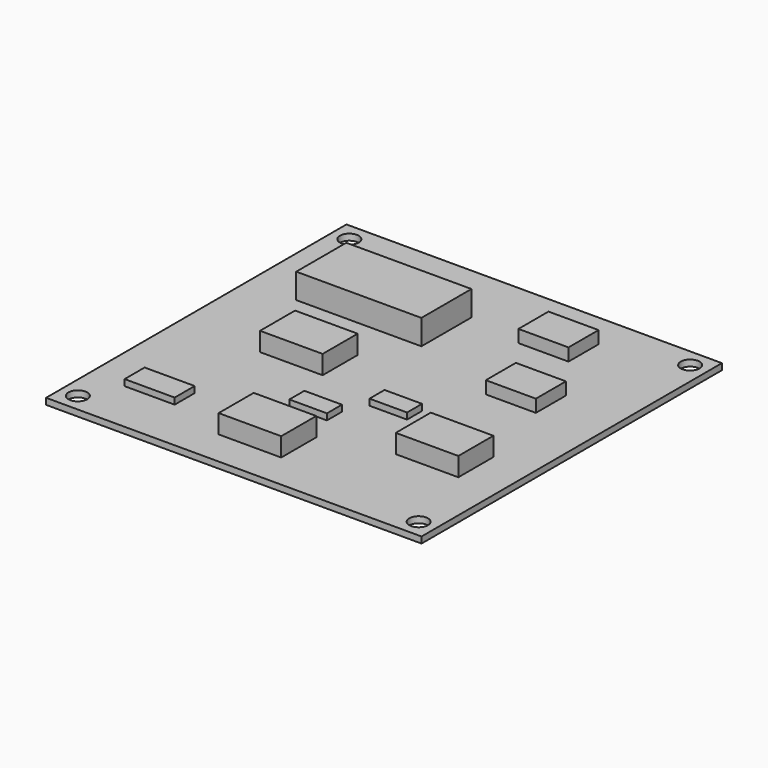
from build123d import *

# Parameters (mm, degrees)
F0_W      = 4
F0_H      = 2
F0_W_2    = 5
F0_H_2    = 3.5
F0_W_3    = 3
F0_H_3    = 1.5
F0_R      = 0.75
F0_W_4    = 10
F0_H_4    = 5
F0_H_5    = 3
F1_DEPTH  = 0.5
F2_DEPTH  = 0.5
F7_DEPTH  = 2
F8_DEPTH  = 1.5
F9_DEPTH  = 1
F10_DEPTH = 0.5


# Not quite as in the source:
# - the program builds the solid bodies; features that only make, move or delete a surface that nothing else refers to are left out


with BuildPart() as f1:
    # F0 (on Top) → F1 (new body)
    with BuildSketch(Plane.XY):
        Polygon((15, 15), (0, 15), (-15, 15), (-15, 0), (-15, -15), (15, -15), (15, 0), align=None)
        with Locations((-10.1540855616, -9.7154753059)):
            Rectangle(F0_W, F0_H, mode=Mode.SUBTRACT)
        with Locations((-1.0007002298, -10.3894498274)):
            Rectangle(F0_W_2, F0_H_2, mode=Mode.SUBTRACT)
        with Locations((-0.9053347297, -5.6935508102)):
            Rectangle(F0_W_3, F0_H_3, mode=Mode.SUBTRACT)
        with Locations((-5.9298439324, -0.0930169439)):
            Rectangle(F0_W_2, F0_H_2, mode=Mode.SUBTRACT)
        with Locations((2.9284434728, -2.4834803706)):
            Rectangle(F0_W_3, F0_H_3, mode=Mode.SUBTRACT)
        with Locations((9.2957332358, -5.5698433965)):
            Rectangle(F0_W_2, F0_H_2, mode=Mode.SUBTRACT)
        with Locations((-13.6142675997, 13.55786765)):
            Circle(F0_R, mode=Mode.SUBTRACT)
        with Locations((-6.0587198287, 7.557784263)):
            Rectangle(F0_W_4, F0_H_4, mode=Mode.SUBTRACT)
        with Locations((8.1385142617, 3.9959300905)):
            Rectangle(F0_W, F0_H_5, mode=Mode.SUBTRACT)
        with Locations((5.4001008607, 10.6776582673)):
            Rectangle(F0_W, F0_H_5, mode=Mode.SUBTRACT)
        with Locations((-6.0587198287, 7.557784263)):
            Rectangle(F0_W_4, F0_H_4)
        with Locations((-5.9298439324, -0.0930169439)):
            Rectangle(F0_W_2, F0_H_2)
        with Locations((-10.1540855616, -9.7154753059)):
            Rectangle(F0_W, F0_H)
        with Locations((-1.0007002298, -10.3894498274)):
            Rectangle(F0_W_2, F0_H_2)
        with Locations((-0.9053347297, -5.6935508102)):
            Rectangle(F0_W_3, F0_H_3)
        with Locations((2.9284434728, -2.4834803706)):
            Rectangle(F0_W_3, F0_H_3)
        with Locations((9.2957332358, -5.5698433965)):
            Rectangle(F0_W_2, F0_H_2)
        with Locations((8.1385142617, 3.9959300905)):
            Rectangle(F0_W, F0_H_5)
        with Locations((5.4001008607, 10.6776582673)):
            Rectangle(F0_W, F0_H_5)
    extrude(amount=-F1_DEPTH)


with BuildPart() as f2:
    # F0 (on Top) → F2 (new body, through all)
    with BuildSketch(Plane.XY):
        with Locations((-13.6142675997, 13.55786765)):
            Circle(F0_R)
    extrude(amount=-F2_DEPTH)


with BuildPart() as f3_1:
    # F3: instance of F2
    add(f2.part.mirror(Plane.XZ))


with BuildPart() as f4_1:
    # F4: instance of F2
    add(f2.part.mirror(Plane.YZ))


with BuildPart() as f4_2:
    # F4: instance of F3_1
    add(f3_1.part.mirror(Plane.YZ))


with BuildPart() as f1_1:
    add(f1.part)

    # F5: cut F3_1, F4_1, F4_2
    add(f3_1.part, mode=Mode.SUBTRACT)
    add(f4_1.part, mode=Mode.SUBTRACT)
    add(f4_2.part, mode=Mode.SUBTRACT)


with BuildPart() as f7:
    # F0 (on Top) → F7 (new body)
    with BuildSketch(Plane.XY):
        with Locations((-6.0587198287, 7.557784263)):
            Rectangle(F0_W_4, F0_H_4)
    extrude(amount=F7_DEPTH)


with BuildPart() as f8:
    # F0 (on Top) → F8 (new body)
    with BuildSketch(Plane.XY):
        with Locations((-5.9298439324, -0.0930169439)):
            Rectangle(F0_W_2, F0_H_2)
    extrude(amount=F8_DEPTH)


with BuildPart() as f8b:
    # F0 (on Top) → F8, piece 2 (new body)
    with BuildSketch(Plane.XY):
        with Locations((-1.0007002298, -10.3894498274)):
            Rectangle(F0_W_2, F0_H_2)
    extrude(amount=F8_DEPTH)


with BuildPart() as f8c:
    # F0 (on Top) → F8, piece 3 (new body)
    with BuildSketch(Plane.XY):
        with Locations((9.2957332358, -5.5698433965)):
            Rectangle(F0_W_2, F0_H_2)
    extrude(amount=F8_DEPTH)


with BuildPart() as f9:
    # F0 (on Top) → F9 (new body)
    with BuildSketch(Plane.XY):
        with Locations((8.1385142617, 3.9959300905)):
            Rectangle(F0_W, F0_H_5)
    extrude(amount=F9_DEPTH)


with BuildPart() as f9b:
    # F0 (on Top) → F9, piece 2 (new body)
    with BuildSketch(Plane.XY):
        with Locations((5.4001008607, 10.6776582673)):
            Rectangle(F0_W, F0_H_5)
    extrude(amount=F9_DEPTH)


with BuildPart() as f10:
    # F0 (on Top) → F10 (new body)
    with BuildSketch(Plane.XY):
        with Locations((-0.9053347297, -5.6935508102)):
            Rectangle(F0_W_3, F0_H_3)
    extrude(amount=F10_DEPTH)


with BuildPart() as f10b:
    # F0 (on Top) → F10, piece 2 (new body)
    with BuildSketch(Plane.XY):
        with Locations((2.9284434728, -2.4834803706)):
            Rectangle(F0_W_3, F0_H_3)
    extrude(amount=F10_DEPTH)


with BuildPart() as f10c:
    # F0 (on Top) → F10, piece 3 (new body)
    with BuildSketch(Plane.XY):
        with Locations((-10.1540855616, -9.7154753059)):
            Rectangle(F0_W, F0_H)
    extrude(amount=F10_DEPTH)


solid = Compound([f1_1.part, f7.part, f8.part, f8b.part, f8c.part, f9.part, f9b.part, f10.part, f10b.part, f10c.part])
